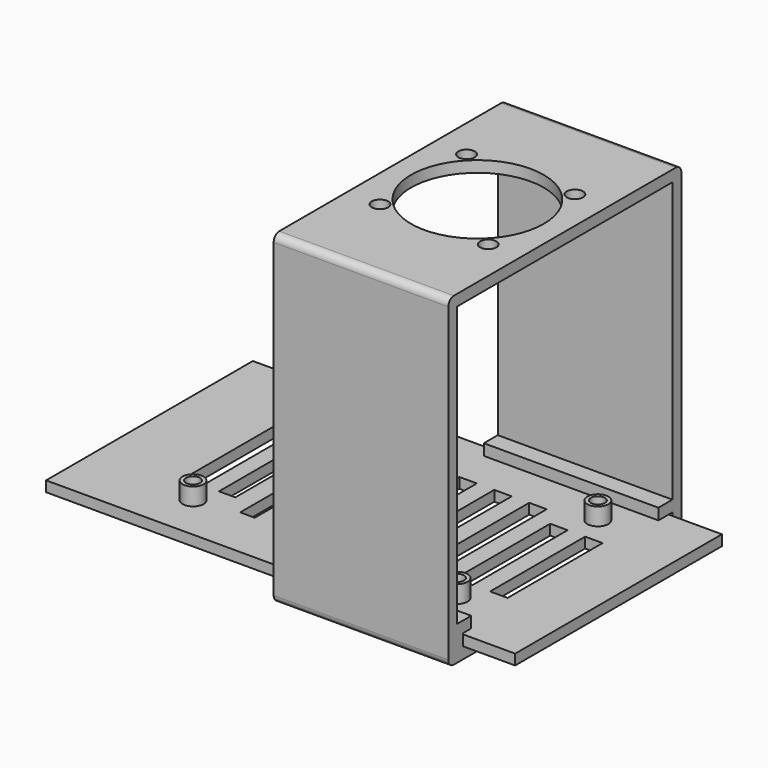
from build123d import *
from build123d import SkipClean  # not in build123d's __all__

# Parameters (mm, degrees)
F0_W      = 134.3
F0_H      = 74
F0_R      = 2
F1_DEPTH  = 3
F2_DEPTH  = 25
F3_R      = 3
F3_R_2    = 2
F4_DEPTH  = 5
F7_W      = 5
F7_H      = 34
F7_H_2    = 44
F7_W_2    = 4.1724147481
F7_W_3    = 4.6632857585
F7_H_3    = 39
F7_W_4    = 5.3995953176
F8_DEPTH  = 25
F10_DEPTH = 50
F11_R     = 2.3384592634
F11_R_2   = 19
F12_DEPTH = 25
F13_R     = 2


# Not quite as in the source:
# - after a boolean that leaves OpenCascade's solid faulty, fix() repairs it
# - a feature names something its author has since deleted; it is built from what else it names


with BuildPart() as f1:
    # F0 (on Top) → F1 (new body)
    with BuildSketch(Plane.XY):
        with Locations((-2.35, 0)):
            Rectangle(F0_W, F0_H)
        with BuildLine():
            Line((-49.5, 22.5), (-46.5, 27))
            Line((-46.5, 27), (-44.7245493689, 27))
            ThreePointArc((-44.7245493689, 27), (-44.1, 27.1000162933), (-43.4754506311, 27))
            Line((-43.4754506311, 27), (48, 27))
            Line((48, 27), (48, 23.31))
            Line((48, 23.31), (49.6, 23.31))
            Line((49.6, 23.31), (49.6, 14.31))
            Line((49.6, 14.31), (48, 14.31))
            Line((48, 14.31), (48, -5.37))
            Line((48, -5.37), (54.8, -5.37))
            Line((54.8, -5.37), (54.8, -17.5))
            Line((54.8, -17.5), (48, -17.5))
            Line((48, -17.5), (48, -27))
            Line((48, -27), (-46.75, -27))
            Line((-46.75, -27), (-46.75, -14.5))
            Line((-46.75, -14.5), (-49.5, -14.5))
            Line((-49.5, -14.5), (-49.5, 22.5))
        make_face(mode=Mode.SUBTRACT)
        with BuildLine():
            Line((-44.7245493689, 27), (-46.5, 27))
            Line((-46.5, 27), (-49.5, 22.5))
            Line((-49.5, 22.5), (-49.5, -14.5))
            Line((-49.5, -14.5), (-46.75, -14.5))
            Line((-46.75, -14.5), (-46.75, -27))
            Line((-46.75, -27), (48, -27))
            Line((48, -27), (48, -17.5))
            Line((48, -17.5), (54.8, -17.5))
            Line((54.8, -17.5), (54.8, -5.37))
            Line((54.8, -5.37), (48, -5.37))
            Line((48, -5.37), (48, 14.31))
            Line((48, 14.31), (49.6, 14.31))
            Line((49.6, 14.31), (49.6, 23.31))
            Line((49.6, 23.31), (48, 23.31))
            Line((48, 23.31), (48, 27))
            Line((48, 27), (-43.4754506311, 27))
            ThreePointArc((-43.4754506311, 27), (-42.4799538991, 26.2728123672), (-42.1, 25.1000162933))
            ThreePointArc((-42.1, 25.1000162933), (-45.272796074, 23.4799701924), (-44.7245493689, 27))
        make_face()
        with Locations((-37.82, -24)):
            Circle(F0_R, mode=Mode.SUBTRACT)
        with Locations((-13.4690740741, -7.7952196389)):
            Circle(F0_R, mode=Mode.SUBTRACT)
        with Locations((37.78, -24)):
            Circle(F0_R, mode=Mode.SUBTRACT)
        with Locations((-13.5170461553, 17.1474736725)):
            Circle(F0_R, mode=Mode.SUBTRACT)
        with Locations((38.8999233283, 24.9872000806)):
            Circle(F0_R, mode=Mode.SUBTRACT)
    extrude(amount=F1_DEPTH)

    # F0 (on Top) → F2 (cut)
    with BuildSketch(Plane.XY):
        with BuildLine():
            ThreePointArc((-43.4754506311, 27), (-44.1, 27.1000162933), (-44.7245493689, 27))
            Line((-44.7245493689, 27), (-43.4754506311, 27))
        make_face()
        with BuildLine():
            Line((-43.4754506311, 27), (-44.7245493689, 27))
            ThreePointArc((-44.7245493689, 27), (-45.272796074, 23.4799701924), (-42.1, 25.1000162933))
            ThreePointArc((-42.1, 25.1000162933), (-42.4799538991, 26.2728123672), (-43.4754506311, 27))
        make_face()
        with Locations((-13.5170461553, 17.1474736725)):
            Circle(F0_R)
        with Locations((38.8999233283, 24.9872000806)):
            Circle(F0_R)
        with Locations((-13.4690740741, -7.7952196389)):
            Circle(F0_R)
        with Locations((-37.82, -24)):
            Circle(F0_R)
        with Locations((37.78, -24)):
            Circle(F0_R)
    extrude(amount=F2_DEPTH, mode=Mode.SUBTRACT)

    # F3 (on face) → F4 (join)
    with BuildSketch(Plane.XY.offset(3)):
        with Locations((-44.1, 25.1000162933)):
            Circle(F3_R)
        with Locations((-44.1, 25.1000162933)):
            Circle(F3_R_2, mode=Mode.SUBTRACT)
        with Locations((-13.5170461553, 17.1474736725)):
            Circle(F3_R)
        with Locations((-13.5170461553, 17.1474736725)):
            Circle(F3_R_2, mode=Mode.SUBTRACT)
        with Locations((38.8999233283, 24.9872000806)):
            Circle(F3_R)
        with Locations((38.8999233283, 24.9872000806)):
            Circle(F3_R_2, mode=Mode.SUBTRACT)
        with Locations((-13.4690740741, -7.7952196389)):
            Circle(F3_R)
        with Locations((-13.4690740741, -7.7952196389)):
            Circle(F3_R_2, mode=Mode.SUBTRACT)
        with Locations((-37.82, -24)):
            Circle(F3_R)
        with Locations((-37.82, -24)):
            Circle(F3_R_2, mode=Mode.SUBTRACT)
        with Locations((37.78, -24)):
            Circle(F3_R)
        with Locations((37.78, -24)):
            Circle(F3_R_2, mode=Mode.SUBTRACT)
    with SkipClean():  # cleaning this boolean's faces spoils the solid; the shape is the same uncleaned
        extrude(amount=F4_DEPTH)

    # F7 (on face) → F8 (cut)
    with BuildSketch(Plane.XY):
        with Locations((44.1262373328, 0)):
            Rectangle(F7_W, F7_H)
        with Locations((24.1262373328, 0)):
            Rectangle(F7_W, F7_H_2)
        with Locations((14.1262373328, 0)):
            Rectangle(F7_W, F7_H_2)
        with Locations((4.1262373328, 0)):
            Rectangle(F7_W, F7_H_2)
        with Locations((-5.8737626672, 0)):
            Rectangle(F7_W, F7_H_2)
        with Locations((-23.837414466, 0)):
            Rectangle(F7_W_2, F7_H_2)
        with Locations((-33.654858008, 2.5)):
            Rectangle(F7_W_3, F7_H_3)
        with Locations((-43.3495822757, 0)):
            Rectangle(F7_W_4, F7_H)
        with Locations((34.1262373328, 0)):
            Rectangle(F7_W, F7_H)
    extrude(amount=F8_DEPTH, mode=Mode.SUBTRACT)

    add(f1.part.fix(), mode=Mode.REPLACE)


with BuildPart() as f10:
    # F9 (on Right) → F10 (new body)
    with BuildSketch(Plane.YZ):
        Polygon((-27.2502614573, 0), (-37.2502614573, 0), (-37.2502614573, 3.4), (-34.2250296303, 3.4), (-34.2250296303, 6.6), (-39.2250296303, 6.6), (-39.2250296303, 86.6), (37.7749703697, 86.6), (37.7749703697, 6.6), (32.7749703697, 6.6), (32.7749703697, 3.4), (37.7749703697, 3.4), (37.7749703697, 0), (27.7749703697, 0), (27.7749703697, -3.2), (40.9749703697, -3.2), (40.9749703697, 89.8), (-42.4250296303, 89.8), (-42.4250296303, -3.2), (-27.2502614573, -3.2), align=None)
    extrude(amount=F10_DEPTH)

    # F11 (on face) → F12 (cut)
    with BuildSketch(Plane.XY.offset(89.8)):
        with Locations((9.4750071671, -16.2250296303)):
            Circle(F11_R)
        with Locations((24.9750071671, -0.7250296303)):
            Circle(F11_R_2)
        with Locations((9.4750071671, 14.7749703697)):
            Circle(F11_R)
        with Locations((40.4750071671, 14.7749703697)):
            Circle(F11_R)
        with Locations((40.4750071671, -16.2250296303)):
            Circle(F11_R)
    extrude(amount=-F12_DEPTH, mode=Mode.SUBTRACT)

    # F13
    f13_edges = [f10.edges().sort_by_distance(p)[0] for p in [
        (25, 40.97497, -3.2),
        (25, -42.42503, -3.2),
        (25, 40.97497, 89.8),
        (25, -42.42503, 89.8),
    ]]
    fillet(f13_edges, radius=F13_R)


solid = Compound([f1.part, f10.part])
